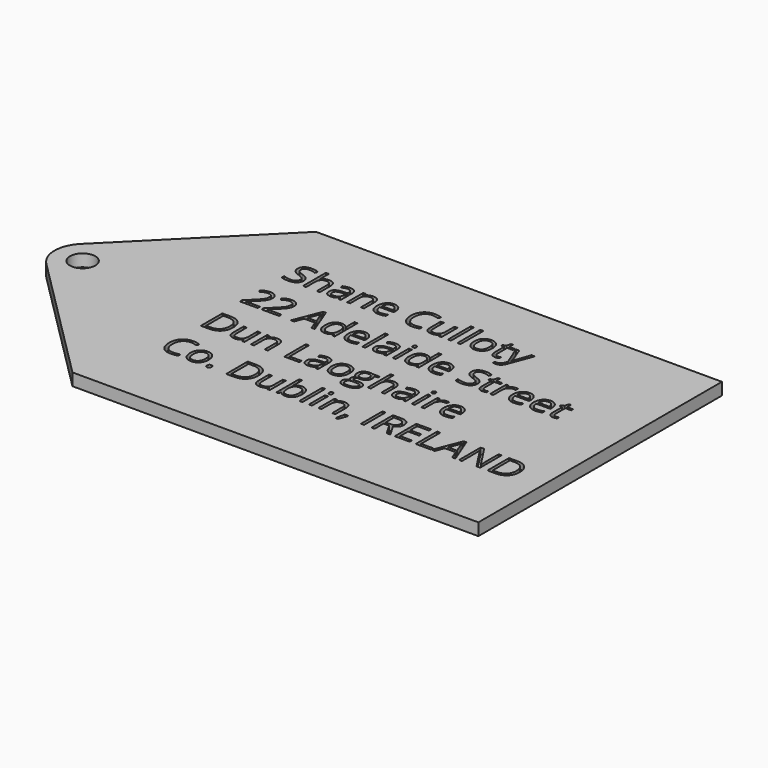
from build123d import *

# Parameters (mm, degrees)
F0_R         = 2.5
F0_W         = 80
F0_H         = 60
F1_DEPTH     = 2.4
F2_TEXT_SIZE = 7.4209044227
F3_DEPTH     = 1.2


# Not quite as in the source:
# - Text() gives the source's letters only with a copy of the font that has no kerning and outlines rounded to 1/6400 em; it was checked with that copy


with BuildPart() as f1:
    # F0 (on Top) → F1 (new body)
    with BuildSketch(Plane.XY):
        with BuildLine():
            Line((-23.865801543, -30), (-23.865801543, 30))
            Line((-23.865801543, 30), (-49.6231608559, 4.2426406871))
            ThreePointArc((-49.6231608559, 4.2426406871), (-51.3805201688, 0), (-49.6231608559, -4.2426406871))
            Line((-49.6231608559, -4.2426406871), (-23.865801543, -30))
        make_face()
        with Locations((-45.865801543, 0)):
            Circle(F0_R, mode=Mode.SUBTRACT)
        with Locations((16.134198457, 0)):
            Rectangle(F0_W, F0_H)
    extrude(amount=F1_DEPTH)

    # F2 (on face) → F3 (cut)
    with BuildSketch(Plane.XY.offset(2.4)):
        with Locations((-18.865801543, 14.6569488156)):
            Text('Shane Culloty', F2_TEXT_SIZE, font='Open Sans', text_align=(TextAlign.LEFT, TextAlign.BOTTOM))
        with Locations((-18.865801543, 4.5645188007)):
            Text('22 Adelaide Street', F2_TEXT_SIZE, font='Open Sans', text_align=(TextAlign.LEFT, TextAlign.BOTTOM))
        with Locations((-18.865801543, -5.5279112142)):
            Text('Dun Laoghaire', F2_TEXT_SIZE, font='Open Sans', text_align=(TextAlign.LEFT, TextAlign.BOTTOM))
        with Locations((-18.865801543, -15.6203412291)):
            Text('Co. Dublin, IRELAND', F2_TEXT_SIZE, font='Open Sans', text_align=(TextAlign.LEFT, TextAlign.BOTTOM))
    extrude(amount=-F3_DEPTH, mode=Mode.SUBTRACT)


solid = f1.part
